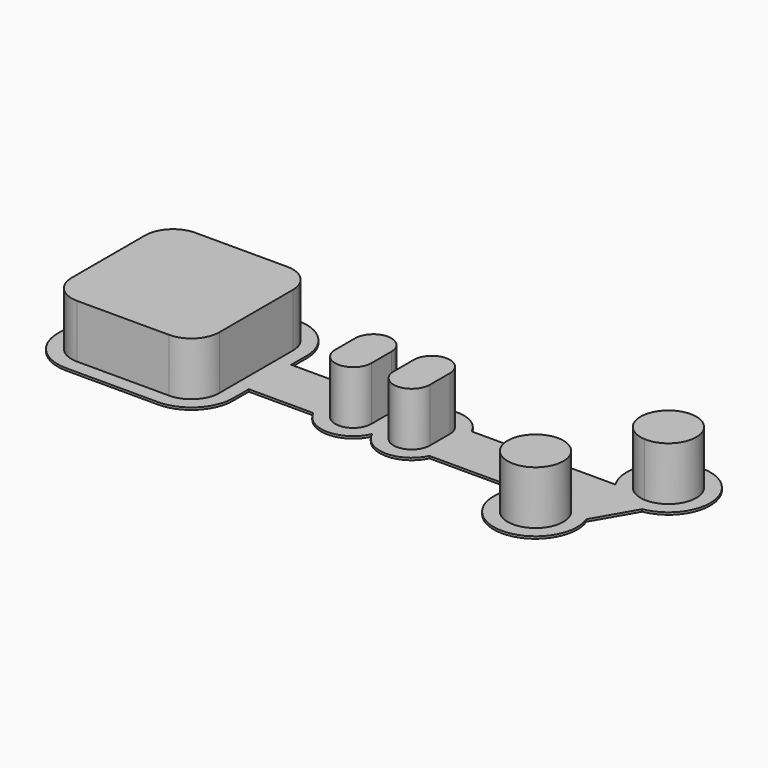
from build123d import *

# Parameters (mm, degrees)
F0_W     = 6.5
F0_H     = 4.5
F0_W_2   = 4
F1_DEPTH = 0.4
F2_DEPTH = 10


with BuildPart() as f1:
    # F0 (on Top) → F1 (new body)
    with BuildSketch(Plane.XY):
        with BuildLine():
            Line((8.25, 15.75), (-8.25, 15.75))
            ThreePointArc((-8.25, 15.75), (-13.5533008589, 13.5533008589), (-15.75, 8.25))
            Line((-15.75, 8.25), (-15.75, -8.25))
            ThreePointArc((-15.75, -8.25), (-13.5533008589, -13.5533008589), (-8.25, -15.75))
            Line((-8.25, -15.75), (8.25, -15.75))
            ThreePointArc((8.25, -15.75), (13.5533008589, -13.5533008589), (15.75, -8.25))
            Line((15.75, -8.25), (15.75, -4.75))
            Line((15.75, -4.75), (27.3219212057, -4.75))
            ThreePointArc((27.3219212057, -4.75), (32.5853423404, -7.9993666334), (37.75, -4.5952078799))
            ThreePointArc((37.75, -4.5952078799), (42.9146576596, -7.9993666334), (48.1780787943, -4.75))
            Line((48.1780787943, -4.75), (63.9480829801, -4.75))
            ThreePointArc((63.9480829801, -4.75), (69.6474451199, -16.1274567319), (77.3637435709, -6.0087617221))
            Line((77.3637435709, -6.0087617221), (81.5596501878, 1.2587617221))
            ThreePointArc((81.5596501878, 1.2587617221), (83.4749132345, 15.4773568118), (73.9480829801, 4.75))
            Line((73.9480829801, 4.75), (48.1780787943, 4.75))
            ThreePointArc((48.1780787943, 4.75), (42.9146576596, 7.9993666334), (37.75, 4.5952078799))
            ThreePointArc((37.75, 4.5952078799), (32.5853423404, 7.9993666334), (27.3219212057, 4.75))
            Line((27.3219212057, 4.75), (15.75, 4.75))
            Line((15.75, 4.75), (15.75, 8.2067806795))
            Line((15.75, 8.2067806795), (15.7488597394, 8.3807769432))
            ThreePointArc((15.7488597394, 8.3807769432), (13.5068608944, 13.5993376728), (8.25, 15.75))
        make_face()
        with BuildLine():
            ThreePointArc((-13.25, 8.25), (-11.7855339059, 11.7855339059), (-8.25, 13.25))
            Line((-8.25, 13.25), (-4.5, 13.25))
            Line((-4.5, 13.25), (4.5, 13.25))
            Line((4.5, 13.25), (8.25, 13.25))
            ThreePointArc((8.25, 13.25), (11.7545739296, 11.8162251152), (13.2492398263, 8.3371846288))
            ThreePointArc((13.2492398263, 8.3371846288), (13.249809953, 8.2935939714), (13.25, 8.25))
            Line((13.25, 8.25), (13.25, 8.2446288243))
            Line((13.25, 8.2446288243), (13.25, 8.2392576486))
            Line((13.25, 8.2392576486), (13.25, 8.2285152972))
            Line((13.25, 8.2285152972), (13.25, 8.2070305943))
            Line((13.25, 8.2070305943), (13.25, 4.5))
            Line((13.25, 4.5), (13.25, 2.25))
            Line((13.25, 2.25), (29.25, 2.25))
            ThreePointArc((29.25, 2.25), (32.5, 5.5), (35.75, 2.25))
            Line((35.75, 2.25), (39.75, 2.25))
            ThreePointArc((39.75, 2.25), (43, 5.5), (46.25, 2.25))
            Line((46.25, 2.25), (72.75, 2.25))
            Line((72.75, 2.25), (74.0490381057, 2.25))
            Line((74.0490381057, 2.25), (76.1669476654, 5.9183269633))
            ThreePointArc((76.1669476654, 5.9183269633), (82.8480762114, 12.9903810568), (80.0640619824, 3.6683269633))
            Line((80.0640619824, 3.6683269633), (74.5292047573, -5.9183269633))
            ThreePointArc((74.5292047573, -5.9183269633), (67.8480762114, -12.9903810568), (70.6320904403, -3.6683269633))
            Line((70.6320904403, -3.6683269633), (71.4509618943, -2.25))
            Line((71.4509618943, -2.25), (46.25, -2.25))
            ThreePointArc((46.25, -2.25), (43, -5.5), (39.75, -2.25))
            Line((39.75, -2.25), (35.75, -2.25))
            ThreePointArc((35.75, -2.25), (32.5, -5.5), (29.25, -2.25))
            Line((29.25, -2.25), (13.25, -2.25))
            Line((13.25, -2.25), (13.25, -4.5))
            Line((13.25, -4.5), (13.25, -8.25))
            ThreePointArc((13.25, -8.25), (11.7855339059, -11.7855339059), (8.25, -13.25))
            Line((8.25, -13.25), (4.5, -13.25))
            Line((4.5, -13.25), (-4.5, -13.25))
            Line((-4.5, -13.25), (-8.25, -13.25))
            ThreePointArc((-8.25, -13.25), (-11.7855339059, -11.7855339059), (-13.25, -8.25))
            Line((-13.25, -8.25), (-13.25, -4.5))
            Line((-13.25, -4.5), (-13.25, 4.5))
            Line((-13.25, 4.5), (-13.25, 8.25))
        make_face(mode=Mode.SUBTRACT)
        Polygon((72.75, 2.25), (46.25, 2.25), (46.25, -2.25), (71.4509618943, -2.25), (74.0490381057, 2.25), align=None)
        Polygon((4.5, 13.25), (-4.5, 13.25), (-4.5, 4.5), (0, 4.5), (4.5, 4.5), align=None)
        Polygon((4.5, -4.5), (0, -4.5), (-4.5, -4.5), (-4.5, -13.25), (4.5, -13.25), align=None)
        Polygon((-4.5, 0), (-4.5, 4.5), (-13.25, 4.5), (-13.25, -4.5), (-4.5, -4.5), align=None)
        Polygon((13.25, 4.5), (4.5, 4.5), (4.5, 0), (4.5, -4.5), (13.25, -4.5), (13.25, -2.25), (13.25, 0), (13.25, 2.25), align=None)
        with BuildLine():
            ThreePointArc((74.5292047573, -5.9183269633), (72.8480762114, -4.3301270189), (70.6320904403, -3.6683269633))
            ThreePointArc((70.6320904403, -3.6683269633), (67.8480762114, -12.9903810568), (74.5292047573, -5.9183269633))
        make_face()
        with BuildLine():
            ThreePointArc((80.0640619824, 3.6683269633), (82.8480762114, 12.9903810568), (76.1669476654, 5.9183269633))
            ThreePointArc((76.1669476654, 5.9183269633), (77.8480762114, 4.3301270189), (80.0640619824, 3.6683269633))
        make_face()
        Polygon((29.25, 2.25), (13.25, 2.25), (13.25, 0), (13.25, -2.25), (29.25, -2.25), (29.25, 0), align=None)
        with BuildLine():
            Line((-4.5, 13.25), (-8.25, 13.25))
            ThreePointArc((-8.25, 13.25), (-11.7855339059, 11.7855339059), (-13.25, 8.25))
            Line((-13.25, 8.25), (-13.25, 4.5))
            Line((-13.25, 4.5), (-4.5, 4.5))
            Line((-4.5, 4.5), (-4.5, 13.25))
        make_face()
        with BuildLine():
            Line((8.25, 13.25), (4.5, 13.25))
            Line((4.5, 13.25), (4.5, 4.5))
            Line((4.5, 4.5), (13.25, 4.5))
            Line((13.25, 4.5), (13.25, 8.2070305943))
            Line((13.25, 8.2070305943), (13.25, 8.2285152972))
            Line((13.25, 8.2285152972), (13.25, 8.2392576486))
            Line((13.25, 8.2392576486), (13.25, 8.2446288243))
            Line((13.25, 8.2446288243), (13.25, 8.25))
            ThreePointArc((13.25, 8.25), (13.249809953, 8.2935939714), (13.2492398263, 8.3371846288))
            ThreePointArc((13.2492398263, 8.3371846288), (11.7545739296, 11.8162251152), (8.25, 13.25))
        make_face()
        with BuildLine():
            Line((-4.5, -4.5), (-13.25, -4.5))
            Line((-13.25, -4.5), (-13.25, -8.25))
            ThreePointArc((-13.25, -8.25), (-11.7855339059, -11.7855339059), (-8.25, -13.25))
            Line((-8.25, -13.25), (-4.5, -13.25))
            Line((-4.5, -13.25), (-4.5, -4.5))
        make_face()
        with BuildLine():
            Line((13.25, -4.5), (4.5, -4.5))
            Line((4.5, -4.5), (4.5, -13.25))
            Line((4.5, -13.25), (8.25, -13.25))
            ThreePointArc((8.25, -13.25), (11.7855339059, -11.7855339059), (13.25, -8.25))
            Line((13.25, -8.25), (13.25, -4.5))
        make_face()
        with BuildLine():
            ThreePointArc((0, 4.5), (-3.1819805153, 3.1819805153), (-4.5, 0))
            ThreePointArc((-4.5, 0), (-3.1819805153, -3.1819805153), (0, -4.5))
            ThreePointArc((0, -4.5), (3.1819805153, -3.1819805153), (4.5, 0))
            ThreePointArc((4.5, 0), (3.1819805153, 3.1819805153), (0, 4.5))
        make_face()
        with BuildLine():
            Line((74.0490381057, 2.25), (71.4509618943, -2.25))
            Line((71.4509618943, -2.25), (70.6320904403, -3.6683269633))
            ThreePointArc((70.6320904403, -3.6683269633), (72.8480762114, -4.3301270189), (74.5292047573, -5.9183269633))
            Line((74.5292047573, -5.9183269633), (80.0640619824, 3.6683269633))
            ThreePointArc((80.0640619824, 3.6683269633), (77.8480762114, 4.3301270189), (76.1669476654, 5.9183269633))
            Line((76.1669476654, 5.9183269633), (74.0490381057, 2.25))
        make_face()
        with Locations((43, 0)):
            Rectangle(F0_W, F0_H)
        Polygon((35.75, 2.25), (29.25, 2.25), (29.25, 0), (29.25, -2.25), (35.75, -2.25), align=None)
        with Locations((37.75, 0)):
            Rectangle(F0_W_2, F0_H)
        with BuildLine():
            ThreePointArc((35.75, 2.25), (32.5, 5.5), (29.25, 2.25))
            Line((29.25, 2.25), (35.75, 2.25))
        make_face()
        with BuildLine():
            Line((35.75, -2.25), (29.25, -2.25))
            ThreePointArc((29.25, -2.25), (32.5, -5.5), (35.75, -2.25))
        make_face()
        with BuildLine():
            Line((46.25, -2.25), (39.75, -2.25))
            ThreePointArc((39.75, -2.25), (43, -5.5), (46.25, -2.25))
        make_face()
        with BuildLine():
            ThreePointArc((46.25, 2.25), (43, 5.5), (39.75, 2.25))
            Line((39.75, 2.25), (46.25, 2.25))
        make_face()
        with BuildLine():
            ThreePointArc((0, -4.5), (-3.1819805153, -3.1819805153), (-4.5, 0))
            Line((-4.5, 0), (-4.5, -4.5))
            Line((-4.5, -4.5), (0, -4.5))
        make_face()
        with BuildLine():
            Line((0, 4.5), (-4.5, 4.5))
            Line((-4.5, 4.5), (-4.5, 0))
            ThreePointArc((-4.5, 0), (-3.1819805153, 3.1819805153), (0, 4.5))
        make_face()
        with BuildLine():
            Line((4.5, -4.5), (4.5, 0))
            ThreePointArc((4.5, 0), (3.1819805153, -3.1819805153), (0, -4.5))
            Line((0, -4.5), (4.5, -4.5))
        make_face()
        with BuildLine():
            Line((4.5, 0), (4.5, 4.5))
            Line((4.5, 4.5), (0, 4.5))
            ThreePointArc((0, 4.5), (3.1819805153, 3.1819805153), (4.5, 0))
        make_face()
    extrude(amount=F1_DEPTH)

    # F0 (on Top) → F2 (join)
    with BuildSketch(Plane.XY):
        with BuildLine():
            Line((-4.5, 13.25), (-8.25, 13.25))
            ThreePointArc((-8.25, 13.25), (-11.7855339059, 11.7855339059), (-13.25, 8.25))
            Line((-13.25, 8.25), (-13.25, 4.5))
            Line((-13.25, 4.5), (-4.5, 4.5))
            Line((-4.5, 4.5), (-4.5, 13.25))
        make_face()
        Polygon((4.5, 13.25), (-4.5, 13.25), (-4.5, 4.5), (0, 4.5), (4.5, 4.5), align=None)
        with BuildLine():
            Line((8.25, 13.25), (4.5, 13.25))
            Line((4.5, 13.25), (4.5, 4.5))
            Line((4.5, 4.5), (13.25, 4.5))
            Line((13.25, 4.5), (13.25, 8.2070305943))
            Line((13.25, 8.2070305943), (13.25, 8.2285152972))
            Line((13.25, 8.2285152972), (13.25, 8.2392576486))
            Line((13.25, 8.2392576486), (13.25, 8.2446288243))
            Line((13.25, 8.2446288243), (13.25, 8.25))
            ThreePointArc((13.25, 8.25), (13.249809953, 8.2935939714), (13.2492398263, 8.3371846288))
            ThreePointArc((13.2492398263, 8.3371846288), (11.7545739296, 11.8162251152), (8.25, 13.25))
        make_face()
        with BuildLine():
            Line((0, 4.5), (-4.5, 4.5))
            Line((-4.5, 4.5), (-4.5, 0))
            ThreePointArc((-4.5, 0), (-3.1819805153, 3.1819805153), (0, 4.5))
        make_face()
        Polygon((-4.5, 0), (-4.5, 4.5), (-13.25, 4.5), (-13.25, -4.5), (-4.5, -4.5), align=None)
        Polygon((13.25, 4.5), (4.5, 4.5), (4.5, 0), (4.5, -4.5), (13.25, -4.5), (13.25, -2.25), (13.25, 0), (13.25, 2.25), align=None)
        with BuildLine():
            Line((4.5, 0), (4.5, 4.5))
            Line((4.5, 4.5), (0, 4.5))
            ThreePointArc((0, 4.5), (3.1819805153, 3.1819805153), (4.5, 0))
        make_face()
        with BuildLine():
            ThreePointArc((0, 4.5), (-3.1819805153, 3.1819805153), (-4.5, 0))
            ThreePointArc((-4.5, 0), (-3.1819805153, -3.1819805153), (0, -4.5))
            ThreePointArc((0, -4.5), (3.1819805153, -3.1819805153), (4.5, 0))
            ThreePointArc((4.5, 0), (3.1819805153, 3.1819805153), (0, 4.5))
        make_face()
        with BuildLine():
            ThreePointArc((0, -4.5), (-3.1819805153, -3.1819805153), (-4.5, 0))
            Line((-4.5, 0), (-4.5, -4.5))
            Line((-4.5, -4.5), (0, -4.5))
        make_face()
        with BuildLine():
            Line((-4.5, -4.5), (-13.25, -4.5))
            Line((-13.25, -4.5), (-13.25, -8.25))
            ThreePointArc((-13.25, -8.25), (-11.7855339059, -11.7855339059), (-8.25, -13.25))
            Line((-8.25, -13.25), (-4.5, -13.25))
            Line((-4.5, -13.25), (-4.5, -4.5))
        make_face()
        with BuildLine():
            Line((4.5, -4.5), (4.5, 0))
            ThreePointArc((4.5, 0), (3.1819805153, -3.1819805153), (0, -4.5))
            Line((0, -4.5), (4.5, -4.5))
        make_face()
        Polygon((4.5, -4.5), (0, -4.5), (-4.5, -4.5), (-4.5, -13.25), (4.5, -13.25), align=None)
        with BuildLine():
            Line((13.25, -4.5), (4.5, -4.5))
            Line((4.5, -4.5), (4.5, -13.25))
            Line((4.5, -13.25), (8.25, -13.25))
            ThreePointArc((8.25, -13.25), (11.7855339059, -11.7855339059), (13.25, -8.25))
            Line((13.25, -8.25), (13.25, -4.5))
        make_face()
        Polygon((35.75, 2.25), (29.25, 2.25), (29.25, 0), (29.25, -2.25), (35.75, -2.25), align=None)
        with BuildLine():
            ThreePointArc((35.75, 2.25), (32.5, 5.5), (29.25, 2.25))
            Line((29.25, 2.25), (35.75, 2.25))
        make_face()
        with BuildLine():
            Line((35.75, -2.25), (29.25, -2.25))
            ThreePointArc((29.25, -2.25), (32.5, -5.5), (35.75, -2.25))
        make_face()
        with Locations((43, 0)):
            Rectangle(F0_W, F0_H)
        with BuildLine():
            ThreePointArc((46.25, 2.25), (43, 5.5), (39.75, 2.25))
            Line((39.75, 2.25), (46.25, 2.25))
        make_face()
        with BuildLine():
            Line((46.25, -2.25), (39.75, -2.25))
            ThreePointArc((39.75, -2.25), (43, -5.5), (46.25, -2.25))
        make_face()
        with BuildLine():
            ThreePointArc((74.5292047573, -5.9183269633), (72.8480762114, -4.3301270189), (70.6320904403, -3.6683269633))
            ThreePointArc((70.6320904403, -3.6683269633), (67.8480762114, -12.9903810568), (74.5292047573, -5.9183269633))
        make_face()
        with BuildLine():
            ThreePointArc((80.0640619824, 3.6683269633), (82.8480762114, 12.9903810568), (76.1669476654, 5.9183269633))
            ThreePointArc((76.1669476654, 5.9183269633), (77.8480762114, 4.3301270189), (80.0640619824, 3.6683269633))
        make_face()
    extrude(amount=F2_DEPTH)


solid = f1.part
